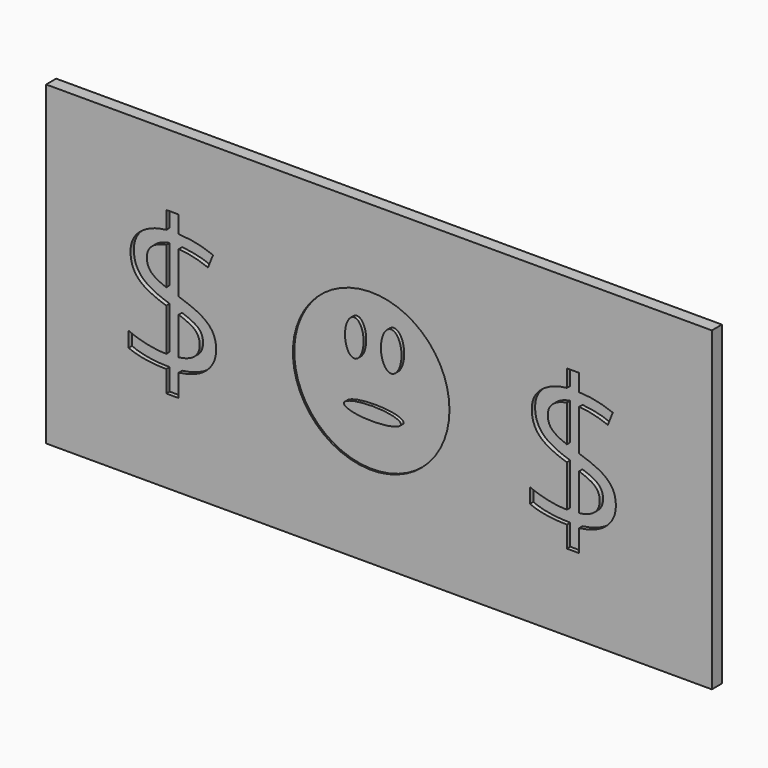
from build123d import *

# Parameters (mm, degrees)
F0_W         = 100.4276946187
F0_H         = 47.673849389
F1_DEPTH     = 1.905
F2_TEXT_SIZE = 29.8504277857
F3_TEXT_SIZE = 29.3076943813
F4_DEPTH     = 0.635
F5_R         = 11.8090567418
F6_DEPTH     = 0.254
F8_DEPTH     = 0.508


# Not quite as in the source:
# - Text() gives the source's letters only with a copy of the font that has no kerning and outlines rounded to 1/6400 em; it was checked with that copy


with BuildPart() as f1:
    # F0 (on Front) → F1 (new body)
    with BuildSketch(Plane.XZ):
        with Locations((-2.0515397191, -0.3907689825)):
            Rectangle(F0_W, F0_H)
    extrude(amount=F1_DEPTH)

    # F2 (on face) + F3 (on face) → F4 (cut)
    with BuildSketch(Plane.XZ.offset(1.905)):
        with Locations((-41.7146161199, -9.9646151066)):
            Text('$', F2_TEXT_SIZE, font='Open Sans', text_align=(TextAlign.LEFT, TextAlign.BOTTOM))
    with BuildSketch(Plane.XZ.offset(1.905)):
        with Locations((18.8546162099, -10.9415389597)):
            Text('$', F3_TEXT_SIZE, font='Open Sans', text_align=(TextAlign.LEFT, TextAlign.BOTTOM))
    extrude(amount=-F4_DEPTH, mode=Mode.SUBTRACT)

    # F5 (on face) → F6 (cut)
    with BuildSketch(Plane.XZ.offset(1.905)):
        with Locations((-3.2238464337, 0)):
            Circle(F5_R)
    extrude(amount=-F6_DEPTH, mode=Mode.SUBTRACT)

    # F7 (on face) → F8 (join)
    with BuildSketch(Plane.XZ.offset(1.651)):
        with BuildLine():
            add(Edge.make_bspline(
                [(-5.5684605613, 2.3446155246), (-3.1432142235, 2.3446155246), (-4.3558373924, 6.4476929838), (-5.5684605613, 10.5507704429), (-6.7810837303, 6.4476929838), (-7.9937068992, 2.3446155246), (-5.5684605613, 2.3446155246)],
                knots=[0, 0, 0, 2.0943951024, 2.0943951024, 4.1887902048, 4.1887902048, 6.2831853072, 6.2831853072, 6.2831853072], degree=2, weights=[1, 0.5, 1, 0.5, 1, 0.5, 1]))
        make_face()
        with BuildLine():
            add(Edge.make_bspline(
                [(0, 2.1492308006), (2.6920834923, 2.1492308006), (1.3460417461, 6.5453853458), (0, 10.9415398911), (-1.3460417461, 6.5453853458), (-2.6920834923, 2.1492308006), (0, 2.1492308006)],
                knots=[0, 0, 0, 2.0943951024, 2.0943951024, 4.1887902048, 4.1887902048, 6.2831853072, 6.2831853072, 6.2831853072], degree=2, weights=[1, 0.5, 1, 0.5, 1, 0.5, 1]))
        make_face()
        with BuildLine():
            add(Edge.make_bspline(
                [(1.4653846156, -4.1030771099), (1.4653846156, -2.3482383867), (-4.9823056906, -3.2256577483), (-11.4299959969, -4.1030771099), (-4.9823056906, -4.9804964715), (1.4653846156, -5.8579158331), (1.4653846156, -4.1030771099)],
                knots=[0, 0, 0, 2.0943951024, 2.0943951024, 4.1887902048, 4.1887902048, 6.2831853072, 6.2831853072, 6.2831853072], degree=2, weights=[1, 0.5, 1, 0.5, 1, 0.5, 1]))
        make_face()
    extrude(amount=F8_DEPTH)


solid = f1.part
